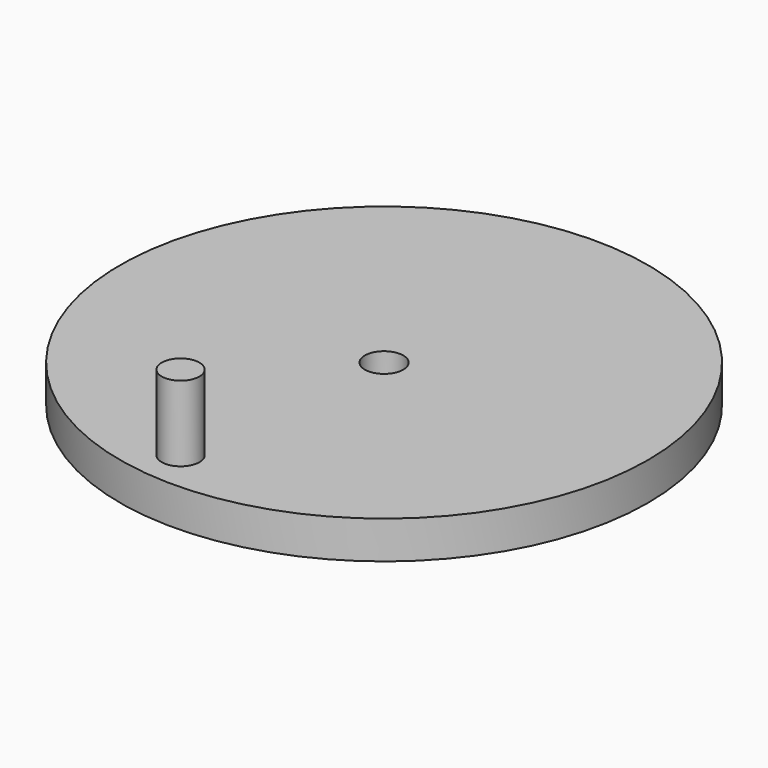
from build123d import *

# Parameters (mm, degrees)
F0_R     = 35
F0_R_2   = 2.55
F1_DEPTH = 5
F2_R     = 2.5
F3_DEPTH = 10


# Not quite as in the source:
# - a feature names something its author has since deleted; it is built from what else it names


with BuildPart() as f1:
    # F0 (on Top) → F1 (new body)
    with BuildSketch(Plane.XY):
        Circle(F0_R)
        Circle(F0_R_2, mode=Mode.SUBTRACT)
    extrude(amount=F1_DEPTH)

    # F2 (on face) → F3 (join)
    with BuildSketch(Plane.XY.offset(5)):
        with Locations((-3.4719216637, -29.3888282031)):
            Circle(F2_R)
    extrude(amount=F3_DEPTH)


solid = f1.part
